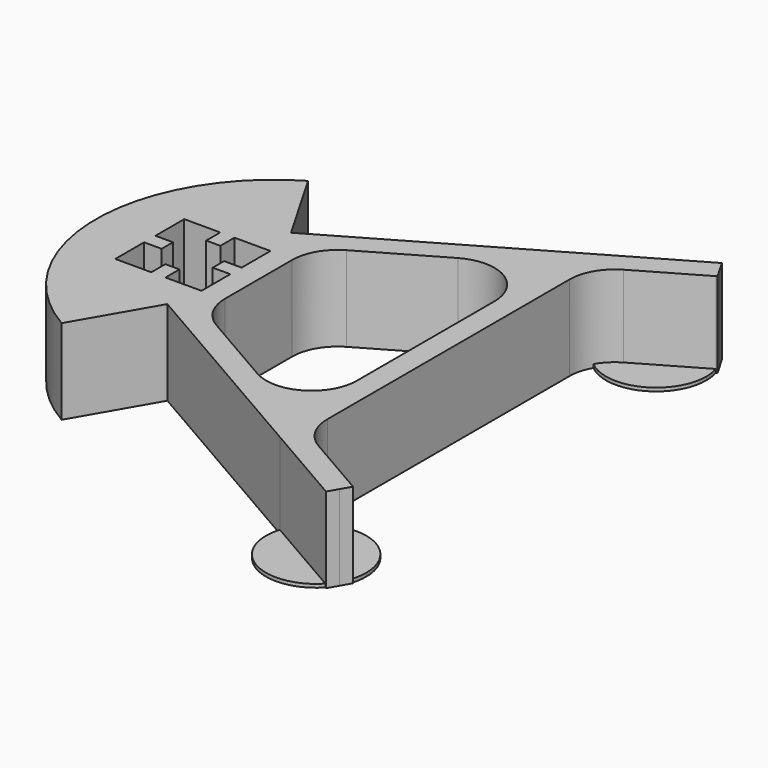
from build123d import *

# Parameters (mm, degrees)
F0_W        = 2.5
F0_H        = 3.1
F0_W_2      = 3.1
F0_H_2      = 2.5
F1_DEPTH    = 15
F2_DEPTH    = 0.6
F3_T1_DEPTH = 15


# Not quite as in the source:
# - a fillet or chamfer that OpenCascade refuses, or shapes differently, is made with other operations: its cross-section is extruded or revolved along the edge and cut away or added


with BuildPart() as f1:
    # F0 (on Top) → F1 (new body)
    with BuildSketch(Plane.XY):
        with BuildLine():
            Line((39.1167589883, 43.6909709372), (38.9183741482, 43.5764333963))
            ThreePointArc((38.9183741482, 43.5764333963), (39.563732113, 42.8018800146), (40.1167589265, 41.9589202367))
            Line((40.1167589265, 41.9589202367), (39.1167589883, 43.6909709372))
        make_face()
        with BuildLine():
            ThreePointArc((40.1167589265, -41.8145826694), (39.563732113, -42.6575424473), (38.9183741482, -43.432095829))
            Line((38.9183741482, -43.432095829), (39.1167589883, -43.5466333699))
            Line((39.1167589883, -43.5466333699), (40.1167589265, -41.8145826694))
        make_face()
        with BuildLine():
            Line((41.1167589883, 40.226869322), (40.1167589265, 41.9589202367))
            ThreePointArc((40.1167589265, 41.9589202367), (40.5702701762, 41.0585049774), (40.9183741482, 40.1123317812))
            Line((40.9183741482, 40.1123317812), (41.1167589883, 40.226869322))
        make_face()
        with BuildLine():
            Line((41.1167589883, -40.0825317547), (40.9183741482, -39.9679942139))
            ThreePointArc((40.9183741482, -39.9679942139), (40.5702701762, -40.9141674102), (40.1167589265, -41.8145826694))
            Line((40.1167589265, -41.8145826694), (41.1167589883, -40.0825317547))
        make_face()
        with BuildLine():
            Line((38.9183741482, 43.5764333963), (23.9946357527, 34.9602090164))
            ThreePointArc((23.9946357527, 34.9602090164), (24.7962509126, 33.113620668), (25.9946357527, 31.4961074012))
            Line((25.9946357527, 31.4961074012), (40.9183741482, 40.1123317812))
            ThreePointArc((40.9183741482, 40.1123317812), (40.5702701762, 41.0585049774), (40.1167589265, 41.9589202367))
            ThreePointArc((40.1167589265, 41.9589202367), (39.563732113, 42.8018800146), (38.9183741482, 43.5764333963))
        make_face()
        with BuildLine():
            ThreePointArc((25.9946357527, -31.3517698339), (24.7962509126, -32.9692831007), (23.9946357527, -34.8158714491))
            Line((23.9946357527, -34.8158714491), (38.9183741482, -43.432095829))
            ThreePointArc((38.9183741482, -43.432095829), (39.563732113, -42.6575424473), (40.1167589265, -41.8145826694))
            ThreePointArc((40.1167589265, -41.8145826694), (40.5702701762, -40.9141674102), (40.9183741482, -39.9679942139))
            Line((40.9183741482, -39.9679942139), (25.9946357527, -31.3517698339))
        make_face()
        with BuildLine():
            Line((23.9946357527, 34.9602090164), (-12.8447652387, 13.6909709372))
            Line((-12.8447652387, 13.6909709372), (-20.6597652387, 27.2269479983))
            ThreePointArc((-20.6597652387, 27.2269479983), (-36.3375843281, 0.0721687836), (-20.6597652387, -27.082610431))
            Line((-20.6597652387, -27.082610431), (-12.8447652387, -13.5466333699))
            Line((-12.8447652387, -13.5466333699), (23.9946357527, -34.8158714491))
            ThreePointArc((23.9946357527, -34.8158714491), (24.7962509126, -32.9692831007), (25.9946357527, -31.3517698339))
            Line((25.9946357527, -31.3517698339), (25.7962509126, -31.2372322931))
            Line((25.7962509126, -31.2372322931), (25.7962509126, 31.3815698604))
            Line((25.7962509126, 31.3815698604), (25.9946357527, 31.4961074012))
            ThreePointArc((25.9946357527, 31.4961074012), (24.7962509126, 33.113620668), (23.9946357527, 34.9602090164))
        make_face()
        Polygon((-7.648612816, -11.9278312164), (-7.648612816, 12.0721687836), (21.7962509126, 29.0721687836), (21.7962509126, -28.9278312164), align=None, mode=Mode.SUBTRACT)
        Polygon((-17.998612816, 7.6721687836), (-11.648612816, 7.6721687836), (-11.648612816, 1.3221687836), (-11.648612816, -1.1778312164), (-11.648612816, -7.5278312164), (-17.998612816, -7.5278312164), (-20.498612816, -7.5278312164), (-26.848612816, -7.5278312164), (-26.848612816, -1.1778312164), (-26.848612816, 1.3221687836), (-26.848612816, 7.6721687836), (-20.498612816, 7.6721687836), align=None, mode=Mode.SUBTRACT)
        with Locations((-19.248612816, -5.9778312164)):
            Rectangle(F0_W, F0_H)
        with Locations((-13.198612816, 0.0721687836)):
            Rectangle(F0_W_2, F0_H_2)
        with Locations((-19.248612816, 6.1221687836)):
            Rectangle(F0_W, F0_H)
        with Locations((-25.298612816, 0.0721687836)):
            Rectangle(F0_W_2, F0_H_2)
    extrude(amount=F1_DEPTH)

    # F0 (on Top) → F2 (join)
    with BuildSketch(Plane.XY):
        with BuildLine():
            ThreePointArc((38.9183741482, 43.5764333963), (28.0338552197, 45.1965244366), (23.9946357527, 34.9602090164))
            Line((23.9946357527, 34.9602090164), (38.9183741482, 43.5764333963))
        make_face()
        with BuildLine():
            Line((39.1167589883, 43.6909709372), (38.9183741482, 43.5764333963))
            ThreePointArc((38.9183741482, 43.5764333963), (39.563732113, 42.8018800146), (40.1167589265, 41.9589202367))
            Line((40.1167589265, 41.9589202367), (39.1167589883, 43.6909709372))
        make_face()
        with BuildLine():
            Line((38.9183741482, -43.432095829), (23.9946357527, -34.8158714491))
            ThreePointArc((23.9946357527, -34.8158714491), (28.0338552197, -45.0521868693), (38.9183741482, -43.432095829))
        make_face()
        with BuildLine():
            ThreePointArc((40.1167589265, -41.8145826694), (39.563732113, -42.6575424473), (38.9183741482, -43.432095829))
            Line((38.9183741482, -43.432095829), (39.1167589883, -43.5466333699))
            Line((39.1167589883, -43.5466333699), (40.1167589265, -41.8145826694))
        make_face()
        with BuildLine():
            Line((41.1167589883, 40.226869322), (40.1167589265, 41.9589202367))
            ThreePointArc((40.1167589265, 41.9589202367), (40.5702701762, 41.0585049774), (40.9183741482, 40.1123317812))
            Line((40.9183741482, 40.1123317812), (41.1167589883, 40.226869322))
        make_face()
        with BuildLine():
            Line((40.9183741482, 40.1123317812), (25.9946357527, 31.4961074012))
            ThreePointArc((25.9946357527, 31.4961074012), (35.7032074646, 29.3083760539), (41.3018044121, 37.5362703988))
            ThreePointArc((41.3018044121, 37.5362703988), (41.2054217299, 38.8384907155), (40.9183741482, 40.1123317812))
        make_face()
        with BuildLine():
            ThreePointArc((41.3018044121, -37.3919328315), (35.7032074646, -29.1640384866), (25.9946357527, -31.3517698339))
            Line((25.9946357527, -31.3517698339), (40.9183741482, -39.9679942139))
            ThreePointArc((40.9183741482, -39.9679942139), (41.2054217299, -38.6941531482), (41.3018044121, -37.3919328315))
        make_face()
        with BuildLine():
            Line((41.1167589883, -40.0825317547), (40.9183741482, -39.9679942139))
            ThreePointArc((40.9183741482, -39.9679942139), (40.5702701762, -40.9141674102), (40.1167589265, -41.8145826694))
            Line((40.1167589265, -41.8145826694), (41.1167589883, -40.0825317547))
        make_face()
    extrude(amount=F2_DEPTH)

    # F3: fillet of radius 8 on 6 edges, made by hand

    # F3_s2 → F3_t1 (join)
    with BuildSketch(Plane.XY):
        with BuildLine():
            ThreePointArc((-3.648612816, 14.3815698604), (-6.5768160463, 11.4533666301), (-7.648612816, 7.4533666301))
            Line((-7.648612816, 7.4533666301), (-7.648612816, 12.0721687836))
            Line((-7.648612816, 12.0721687836), (-3.648612816, 14.3815698604))
        make_face()
        with BuildLine():
            ThreePointArc((25.7962509126, 26.7627677069), (26.8680476824, 30.7627677069), (29.7962509126, 33.6909709372))
            Line((29.7962509126, 33.6909709372), (25.7962509126, 31.3815698604))
            Line((25.7962509126, 31.3815698604), (25.7962509126, 26.7627677069))
        make_face()
        with BuildLine():
            ThreePointArc((21.7962509126, 15.2157623231), (17.7962509126, 22.1439655534), (9.7962509126, 22.1439655534))
            Line((9.7962509126, 22.1439655534), (21.7962509126, 29.0721687836))
            Line((21.7962509126, 29.0721687836), (21.7962509126, 15.2157623231))
        make_face()
        with BuildLine():
            ThreePointArc((21.7962509126, -15.0714247558), (17.7962509126, -21.9996279861), (9.7962509126, -21.9996279861))
            Line((9.7962509126, -21.9996279861), (21.7962509126, -28.9278312164))
            Line((21.7962509126, -28.9278312164), (21.7962509126, -15.0714247558))
        make_face()
        with BuildLine():
            ThreePointArc((29.7962509126, -33.5466333699), (26.8680476824, -30.6184301396), (25.7962509126, -26.6184301396))
            Line((25.7962509126, -26.6184301396), (25.7962509126, -31.2372322931))
            Line((25.7962509126, -31.2372322931), (29.7962509126, -33.5466333699))
        make_face()
        with BuildLine():
            ThreePointArc((-7.648612816, -7.3090290628), (-6.5768160463, -11.3090290628), (-3.648612816, -14.2372322931))
            Line((-3.648612816, -14.2372322931), (-7.648612816, -11.9278312164))
            Line((-7.648612816, -11.9278312164), (-7.648612816, -7.3090290628))
        make_face()
    extrude(amount=F3_T1_DEPTH)


solid = f1.part
